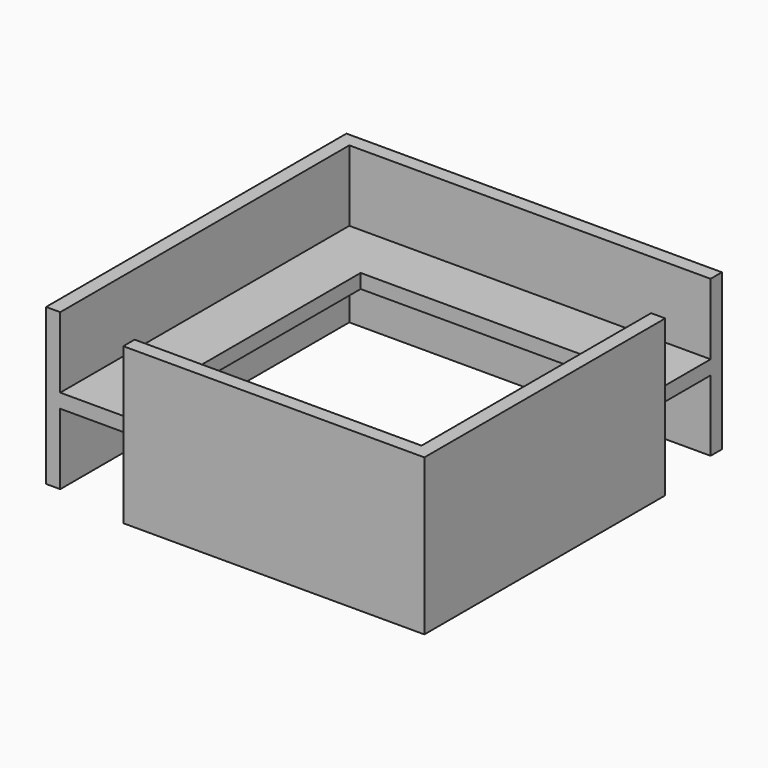
from build123d import *

# Parameters (mm, degrees)
F1_DEPTH = 12
F0_W     = 35
F0_H     = 35
F2_DEPTH = 2
F0_R     = 5
F3_DEPTH = 10


with BuildPart() as f1:
    # F0 (on Top) → F1 (new body)
    with BuildSketch(Plane.XY):
        Polygon((24.28125, 28.71875), (-28.71875, 28.71875), (-28.71875, -24.28125), (-26.71875, -24.28125), (-26.71875, 26.71875), (24.28125, 26.71875), align=None)
    extrude(amount=F1_DEPTH)



with BuildPart() as f1b:
    # F0 (on Top) → F1, piece 2 (new body)
    with BuildSketch(Plane.XY):
        Polygon((26.28125, -26.28125), (26.28125, 16.21875), (24.28125, 16.21875), (24.28125, -24.28125), (-16.21875, -24.28125), (-16.21875, -26.28125), align=None)
    extrude(amount=F1_DEPTH)


with BuildPart() as f1_1:
    add(f1.part)

    add(f1b.part)  # F2 merges F1b
    # F0 (on Top) → F2 (join)
    with BuildSketch(Plane.XY):
        Polygon((24.28125, 18.71875), (24.28125, 26.71875), (-26.71875, 26.71875), (-26.71875, -24.28125), (-18.71875, -24.28125), (-16.21875, -24.28125), (24.28125, -24.28125), (24.28125, 16.21875), align=None)
        with Locations((-1.21875, 1.21875)):
            Rectangle(F0_W, F0_H, mode=Mode.SUBTRACT)
    extrude(amount=F2_DEPTH)

    # F0 (on Top) → F3 (join)
    with BuildSketch(Plane.XY):
        Polygon((24.28125, 28.71875), (-28.71875, 28.71875), (-28.71875, -24.28125), (-26.71875, -24.28125), (-26.71875, 26.71875), (24.28125, 26.71875), align=None)
        Polygon((26.28125, -26.28125), (26.28125, 16.21875), (24.28125, 16.21875), (24.28125, -24.28125), (-16.21875, -24.28125), (-16.21875, -26.28125), align=None)
    extrude(amount=-F3_DEPTH)


with BuildPart() as f2:
    # F0 (on Top) → F2, piece 2 (new body)
    with BuildSketch(Plane.XY):
        with Locations((-1.21875, 1.21875)):
            Circle(F0_R)
    extrude(amount=F2_DEPTH)


solid = f1_1.part
